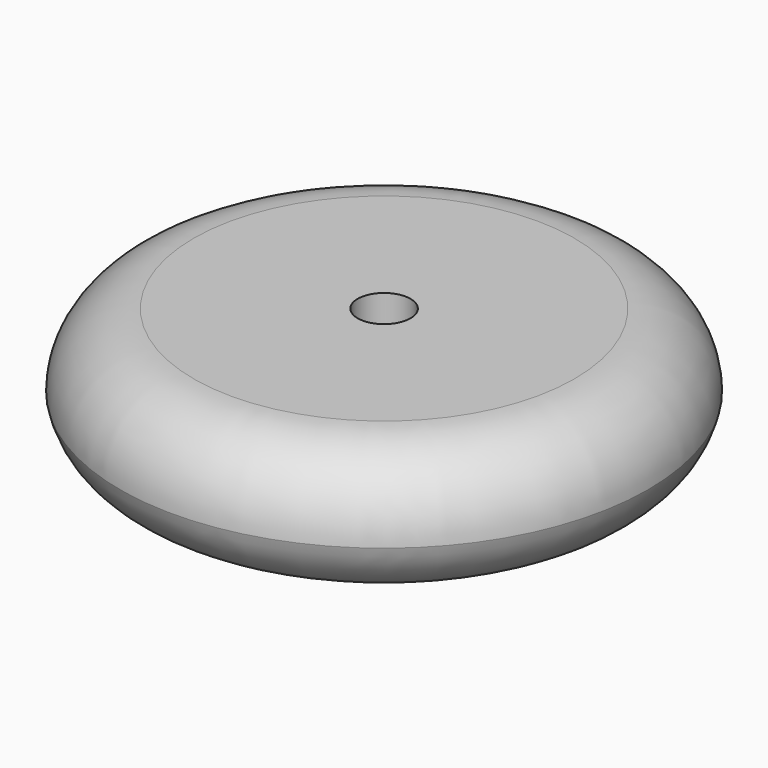
from build123d import *

# Parameters (mm, degrees)
F2_R = 2.7869198521


# Not quite as in the source:
# - a fillet or chamfer that OpenCascade refuses, or shapes differently, is made with other operations: its cross-section is extruded or revolved along the edge and cut away or added


with BuildPart() as f1:
    # F0 (on Front) → F1 (revolve)
    with BuildSketch(Plane.XZ):
        Polygon((8.5, -2.5), (10, -2.5), (10, 2.5), (8.5, 2.5), (1, 2.5), (1, -2.5), align=None)
    revolve(axis=Axis((0, 0, 0), (0, 0, -1)))

    # F2
    f2_edges = [f1.edges().sort_by_distance(p)[0] for p in [
        (-10, 0, 2.5),
    ]]
    fillet(f2_edges, radius=F2_R)

    # F3: fillet of radius 2.787 on 1 edges, made by hand

    # F3_s1 → F3_t2 (revolve, cut)
    with BuildSketch(Plane.XZ):
        with BuildLine():
            ThreePointArc((10, -0.2869198521), (9.0288444344, -1.8771261086), (7.2727330524, -2.5))
            Line((7.2727330524, -2.5), (10, -2.5))
            Line((10, -2.5), (10, -0.2869198521))
        make_face()
    revolve(axis=Axis((0, 0, -2.5), (0, 0, -1)), mode=Mode.SUBTRACT)


solid = f1.part
